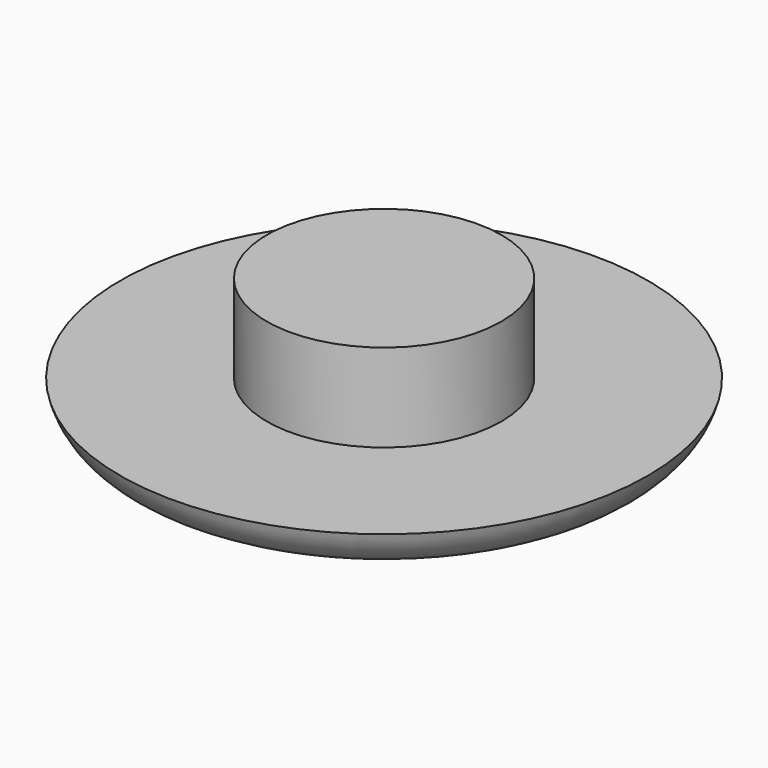
from build123d import *

# Parameters (mm, degrees)
F0_R     = 9
F1_DEPTH = 1.5
F2_R     = 4
F3_DEPTH = 3
F5_R     = 6
F6_DEPTH = 0.25


# Not quite as in the source:
# - a fillet or chamfer that OpenCascade refuses, or shapes differently, is made with other operations: its cross-section is extruded or revolved along the edge and cut away or added


with BuildPart() as f1:
    # F0 (on Top) → F1 (new body)
    with BuildSketch(Plane.XY):
        Circle(F0_R)
    extrude(amount=F1_DEPTH)

    # F2 (on face) → F3 (join)
    with BuildSketch(Plane.XY.offset(1.5)):
        Circle(F2_R)
    extrude(amount=F3_DEPTH)

    # F4: fillet of radius 2 on 1 edges, made by hand

    # F4_s1 → F4_t2 (revolve, cut)
    with BuildSketch(Plane.XZ):
        with BuildLine():
            ThreePointArc((9, 1.5), (8.2882531983, 0.4188611699), (7.0635083269, 0))
            Line((7.0635083269, 0), (9, 0))
            Line((9, 0), (9, 1.5))
        make_face()
    revolve(axis=Axis((0, 0, 0), (0, 0, 1)), mode=Mode.SUBTRACT)

    # F5 (on face) → F6 (cut)
    with BuildSketch(Plane(origin=(0, 0, 0), x_dir=(1, 0, 0), z_dir=(0, 0, -1))):
        Circle(F5_R)
        with BuildLine():
            ThreePointArc((0, 5), (3.5355339059, 3.5355339059), (5, 0))
            ThreePointArc((5, 0), (3.5355339059, -3.5355339059), (0, -5))
            ThreePointArc((0, -5), (-3.5355339059, -3.5355339059), (-5, 0))
            ThreePointArc((-5, 0), (-3.5355339059, 3.5355339059), (0, 5))
        make_face(mode=Mode.SUBTRACT)
    extrude(amount=-F6_DEPTH, mode=Mode.SUBTRACT)


solid = f1.part
